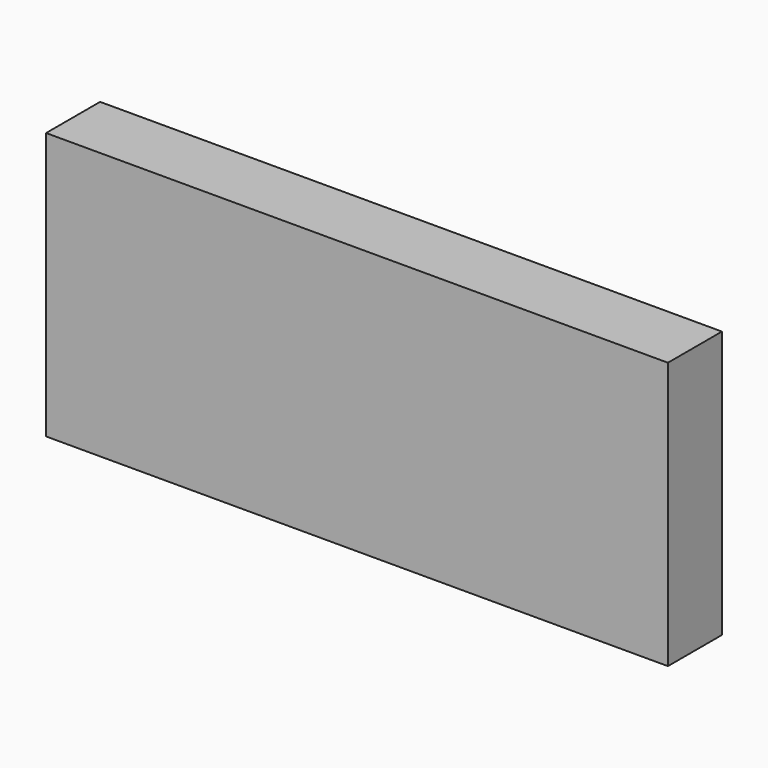
from build123d import *

# Parameters (mm, degrees)
F0_W     = 233.9657619596
F0_H     = 100.5053790286
F1_DEPTH = 25.4


# Not quite as in the source:
# - the program builds the solid bodies; features that only make, move or delete a surface that nothing else refers to are left out


with BuildPart() as f1:
    # F0 (on Front) → F1 (new body)
    with BuildSketch(Plane.XZ):
        with Locations((-79.9240730703, -39.9791090749)):
            Rectangle(F0_W, F0_H)
    extrude(amount=F1_DEPTH)


solid = f1.part
